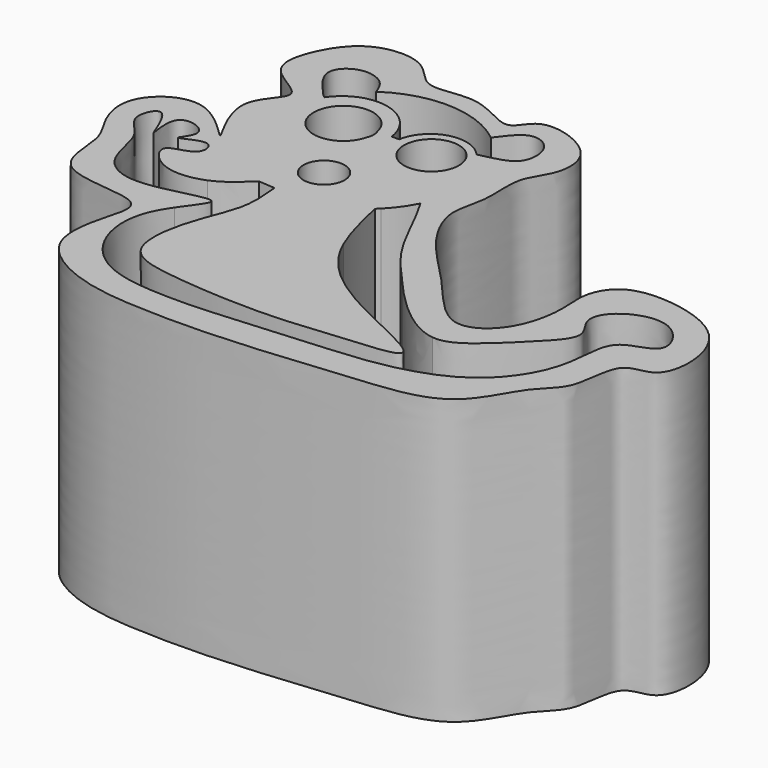
from build123d import *

# Parameters (mm, degrees)
F0_R     = 3.7205580231
F1_DEPTH = 51.562


with BuildPart() as f1:
    # F0 (on Top) → F1 (new body)
    with BuildSketch(Plane.XY):
        with BuildLine():
            add(Edge.make_bspline(
                [(-53.0351996422, 40.0811992586), (-53.3079930687, 41.6627953679), (-60.7647197567, 44.1354743978), (-59.1255177726, 52.4056801186), (-53.9738105286, 59.9405136718), (-43.6820680314, 60.0552836973), (-40.0768432819, 52.8134528274), (-30.922173083, 56.6842073685), (-22.4287718601, 49.6258780063), (-20.555433276, 57.2186201881), (-8.0154700964, 53.1735527396), (-7.9074828777, 44.5223918176), (-12.1257390745, 40.114923321), (-10.7256442044, 31.933104297), (-13.5341011998, 25.6774370624), (-8.5652531319, 16.3662428058), (-0.0531398385, 8.862949751), (8.2077255005, -2.4517748861), (16.5242775456, 2.6540873778), (18.6817624376, 12.0345401673), (17.4626842494, 17.7274123298), (20.6284477431, 24.0450881696), (30.6198326835, 24.2634316934), (39.9883133501, 20.6347344654), (43.274263606, 12.4930502219), (41.8209757823, 4.373088916), (34.4557856792, 5.3826149304), (35.1162405235, -5.4890850104), (29.2679840475, -8.9956139239), (24.7245789247, -21.1012100778), (8.5716456517, -22.3660177487), (-3.2073427267, -23.673208758), (-17.0097819532, -24.6958343574), (-27.8201507989, -24.6594358256), (-40.6695843247, -23.820251083), (-51.9653752301, -17.0200309695), (-50.4154986842, -6.6540089959), (-47.0885578266, 2.3917477436), (-66.4204916011, 0.0746272617), (-65.0768362054, 12.6106814261), (-68.7260787409, 16.8312978332), (-71.4451206704, 25.4892643605), (-60.6602210105, 33.1244068312), (-49.112760512, 18.8797609199), (-59.7521417466, 34.36020266), (-52.7621453219, 38.4980905445), (-53.0351996422, 40.0811992586)],
                knots=[0, 0, 0, 0, 0.0210227239, 0.0415498789, 0.0644000682, 0.0870516541, 0.1064951093, 0.129047416, 0.1514029912, 0.1678357279, 0.1925133649, 0.2131914357, 0.2315774148, 0.2528958574, 0.2725256217, 0.2962058086, 0.3233948157, 0.3502333972, 0.3708847816, 0.3943700022, 0.4129475644, 0.4314604615, 0.4548624528, 0.4788890461, 0.5011629669, 0.5210807734, 0.5382113528, 0.5607203848, 0.5804368125, 0.606432177, 0.6361158369, 0.6634705602, 0.6917741726, 0.7173460798, 0.7451067546, 0.7712430171, 0.7953524467, 0.8146494037, 0.8431599135, 0.8666451338, 0.8851189078, 0.9065051395, 0.9308580695, 0.9545133683, 0.9789571704, 1, 1, 1, 1], degree=3))
        make_face()
        with BuildLine():
            add(Edge.make_bspline(
                [(-21.0652948492, 20.6782598491), (-21.670172812, 20.639156422), (-21.7699233734, 20.2162934835), (-21.7458119728, 20.0338150913)],
                knots=[0.8847102512, 0.8847102512, 0.8847102512, 0.8847102512, 0.9803485, 0.9803485, 0.9803485, 0.9803485], degree=3))
            ThreePointArc((-21.0652948492, 20.6782598491), (-19.1925492315, 22.8925325451), (-17.6995540947, 25.3787234554))
            add(Edge.make_bspline(
                [(-8.1258436749, 8.8725080124), (-8.9507770078, 9.8625538653), (-11.8076923951, 13.5529828734), (-14.9203133764, 20.5039164014), (-16.8647921862, 23.9151210734), (-17.6995540947, 25.3787234554)],
                knots=[0.936730527, 0.936730527, 0.936730527, 0.936730527, 0.948494633, 0.9779000116, 1, 1, 1, 1], degree=3))
            add(Edge.make_bspline(
                [(-8.1258436749, 8.8725080124), (-6.9920288455, 7.5914053785), (-5.8582140161, 6.3103027445), (-4.7243991867, 5.0292001106)],
                knots=[0, 0, 0, 0, 5.1323328258, 5.1323328258, 5.1323328258, 5.1323328258], degree=3))
            add(Edge.make_bspline(
                [(9.2964004725, -5.6388000958), (6.2140361423, -5.3139568809), (-0.4758535739, 0.0377445161), (-3.1854275389, 3.3122390614), (-4.7243991867, 5.0292001106)],
                knots=[0.8640116613, 0.8640116613, 0.8640116613, 0.8640116613, 0.8951731635, 0.9199974846, 0.9199974846, 0.9199974846, 0.9199974846], degree=3))
            add(Edge.make_bspline(
                [(-44.1327011496, 2.6484160648), (-44.7130309574, 1.8048856406), (-47.6946083402, -2.927021188), (-46.8772518965, -11.6007203583), (-39.5802529159, -18.6266633144), (-28.3429017795, -19.591076178), (-18.1242244322, -19.144415426), (-6.9103865804, -18.0520208922), (4.7211664853, -17.4405127728), (13.9368833116, -15.7759420728), (23.8112421331, -11.3932618369), (30.3389740044, -0.7257155667), (28.9709345734, 10.3098746354), (39.2162281551, 10.6255935235), (33.8249627001, 20.1168201293), (24.5686551298, 17.1746113113), (22.2539715483, 11.9137811577), (26.7972968019, 7.9772485427), (21.1542360401, 2.2425014104), (16.0200417627, -2.9179627405), (11.7632185561, -5.8987723219), (9.2964004725, -5.6388000958)],
                knots=[0.3585684754, 0.3585684754, 0.3585684754, 0.3585684754, 0.3659479306, 0.3974689583, 0.4260715846, 0.4571624421, 0.4875914142, 0.5193796367, 0.5515918337, 0.5804502736, 0.6108726721, 0.6438200053, 0.672548465, 0.6962237578, 0.7206702006, 0.748010088, 0.7683723479, 0.7881144061, 0.8123813661, 0.8390730918, 0.8640116613, 0.8640116613, 0.8640116613, 0.8640116613], degree=3))
            add(Edge.make_bspline(
                [(-49.0828990199, 6.1701741385), (-49.177863489, 4.040428207), (-47.197859123, 2.9614294526), (-44.13270115, 2.6484160654)],
                knots=[0.0841406615, 0.0841406615, 0.0841406615, 0.0841406615, 0.208246285, 0.208246285, 0.208246285, 0.208246285], degree=3))
            add(Edge.make_bspline(
                [(-45.71999982, 12.0395999402), (-48.2095024269, 11.0006678158), (-53.7802194274, 10.5093334281), (-58.6217302771, 16.9809530467), (-51.186861328, 16.9659773531), (-52.1172615159, 22.6049918831), (-59.260802502, 17.953520738), (-53.6590125511, 23.3854970332), (-62.6446993243, 26.277051321), (-59.5639044419, 14.4067842249), (-63.6375573492, 27.3151683753), (-66.9947393471, 20.1703294936), (-61.4699964034, 17.1271549744), (-61.3142437426, 8.4281658926), (-55.8384577489, 5.0155903157), (-50.3902321248, 5.8993125354), (-49.0828990199, 6.1701741385)],
                knots=[0.0256288773, 0.0256288773, 0.0256288773, 0.0256288773, 0.0524870758, 0.0732332952, 0.0938749966, 0.1097169476, 0.1296254117, 0.1467479568, 0.1673048843, 0.1888353489, 0.2125106443, 0.2303278097, 0.2524804134, 0.2787225334, 0.3057488565, 0.3143296922, 0.3143296922, 0.3143296922, 0.3143296922], degree=3))
            add(Edge.make_bspline(
                [(-39.7831306216, 16.380742902), (-41.56390775, 14.7159485647), (-43.3444437298, 13.0309793139), (-45.71999982, 12.0395999402)],
                knots=[0, 0, 0, 0, 0.0256288773, 0.0256288773, 0.0256288773, 0.0256288773], degree=3))
            add(Edge.make_bspline(
                [(-39.7831306216, 16.380742902), (-38.95093334, 16.2972918142), (-38.134915658, 16.2371630687), (-37.335459951, 16.2009078471)],
                knots=[0, 0, 0, 0, 2.0774208338, 2.0774208338, 2.0774208338, 2.0774208338], degree=3))
            add(Edge.make_bspline(
                [(-37.335459951, 16.2009078471), (-31.0549759584, 15.916088642), (-25.796629976, 17.1046466153), (-21.7458119642, 20.0338150896)],
                knots=[2.0774208338, 2.0774208338, 2.0774208338, 2.0774208338, 18.3975348551, 18.3975348551, 18.3975348551, 18.3975348551], degree=3))
        make_face(mode=Mode.SUBTRACT)
        with Locations((-34.2900007963, 24.2315996438)):
            Circle(F0_R, mode=Mode.SUBTRACT)
        with BuildLine():
            ThreePointArc((-36.3116717652, 36.4814959466), (-46.971085664, 37.8051259579), (-36.2804545776, 38.8470031321))
            add(Edge.make_bspline(
                [(-36.2804545776, 38.8470031321), (-36.2042632894, 38.638003094), (-36.0421633968, 38.1933474837), (-36.013318579, 37.2966688863), (-36.2123204756, 36.7529476575), (-36.3116717652, 36.4814959466)],
                knots=[0, 0, 0, 0, 0.307532383, 0.6542869592, 1, 1, 1, 1], degree=3))
        make_face(mode=Mode.SUBTRACT)
        with BuildLine():
            ThreePointArc((-20.7269751995, 37.8729701042), (-30.0915433108, 35.5184298259), (-22.954191543, 42.0220600103))
            ThreePointArc((-22.954191543, 42.0220600103), (-21.3189790012, 40.2275103826), (-20.7269751995, 37.8729701042))
        make_face(mode=Mode.SUBTRACT)
        with BuildLine():
            ThreePointArc((-33.7017707591, 38.8470031321), (-39.999476926, 45.7439636175), (-48.6812743523, 42.3007731858))
            add(Edge.make_bspline(
                [(-49.2198829041, 42.7281072575), (-49.0385020241, 42.5844299812), (-48.8626552323, 42.4444504621), (-48.6812743523, 42.3007731858)],
                knots=[0, 0, 0, 0, 0.687541694, 0.687541694, 0.687541694, 0.687541694], degree=3))
            add(Edge.make_bspline(
                [(-49.2198829041, 42.7281072575), (-51.19934658, 44.8979233113), (-54.7239489701, 48.7439745563), (-50.1221749988, 52.81542629), (-45.2801795053, 51.5125545977), (-44.4254927385, 49.2654049663), (-44.0268645913, 48.2185372916)],
                knots=[0, 0, 0, 0, 0.310725073, 0.5499326634, 0.79062154, 1, 1, 1, 1], degree=3))
            ThreePointArc((-44.0268645913, 48.2185372916), (-33.1420930224, 51.3687844299), (-22.5308552567, 47.3933671914))
            add(Edge.make_bspline(
                [(-22.5308552567, 47.3933671914), (-21.2095190932, 49.205980475), (-18.7721682592, 52.552915334), (-13.7470974395, 50.0324472001), (-13.8185248481, 43.9096057901), (-16.9020924696, 43.0581948555), (-18.3954862509, 42.6449623371)],
                knots=[0, 0, 0, 0, 0.2768007406, 0.5090744039, 0.7627286351, 1, 1, 1, 1], degree=3))
            add(Edge.make_bspline(
                [(-18.3954862509, 42.6449623371), (-19.1555240256, 42.4677094098), (-19.9155618003, 42.2904564826), (-20.675599575, 42.1132035553)],
                knots=[0, 0, 0, 0, 2.341299676, 2.341299676, 2.341299676, 2.341299676], degree=3))
            add(Edge.make_bspline(
                [(-20.675599575, 42.1132035553), (-20.7297600417, 42.0839673312), (-20.7802752843, 42.0578559737), (-20.8344357509, 42.0286197495)],
                knots=[0, 0, 0, 0, 0.1799537468, 0.1799537468, 0.1799537468, 0.1799537468], degree=3))
            ThreePointArc((-20.8344357509, 42.0286197495), (-20.8671966944, 42.0665437034), (-20.9002447034, 42.1042177634))
            ThreePointArc((-20.9002447034, 42.1042177634), (-27.6501958711, 44.0808092286), (-32.3487092883, 38.8470031321))
            Line((-32.3487092883, 38.8470031321), (-33.7017707591, 38.8470031321))
        make_face(mode=Mode.SUBTRACT)
        with BuildLine():
            add(Edge.make_bspline(
                [(-38.8865054324, 2.7137341923), (-39.2013483841, 1.8508518548), (-40.6857275806, -2.479034825), (-41.857395368, -12.156175759), (-30.2869064904, -14.3210148671), (-13.4186121607, -15.3017300236), (-1.8057579388, -13.7083720265), (15.1351427548, -12.8048451743), (-7.3018340252, -4.1578341465), (-15.5277854797, 2.920156624), (-18.0961822011, 8.0444989939), (-18.4368261233, 8.8112696576)],
                knots=[0.141118669, 0.141118669, 0.141118669, 0.141118669, 0.1655386981, 0.2585924292, 0.3477026087, 0.4665688636, 0.573696851, 0.6603811929, 0.7756371935, 0.8916603721, 0.9113790023, 0.9113790023, 0.9113790023, 0.9113790023], degree=3))
            add(Edge.make_bspline(
                [(-38.8865054322, 2.7137341917), (-32.1377612072, 3.3669214959), (-23.6097595892, 5.891801251), (-18.4368261233, 8.8112696576)],
                knots=[0.2698570737, 0.2698570737, 0.2698570737, 0.2698570737, 0.4846901848, 0.4846901848, 0.4846901848, 0.4846901848], degree=3))
        make_face()
        with BuildLine():
            add(Edge.make_bspline(
                [(-18.4368261233, 8.8112696576), (-19.9677744688, 12.2573498677), (-20.8431582774, 16.1554617481), (-21.718542086, 20.0535736285)],
                knots=[0.9113790023, 0.9113790023, 0.9113790023, 0.9113790023, 1, 1, 1, 1], degree=3))
            add(Edge.make_bspline(
                [(-21.7458119728, 20.0338150913), (-21.7456147196, 20.0323222517), (-21.7404521603, 19.9952311482), (-21.7301917205, 19.9685048959), (-21.718542086, 20.0535736285)],
                knots=[0.9803485, 0.9803485, 0.9803485, 0.9803485, 0.981130908, 1, 1, 1, 1], degree=3))
            add(Edge.make_bspline(
                [(-37.335459951, 16.2009078471), (-31.0549759584, 15.916088642), (-25.796629976, 17.1046466153), (-21.7458119642, 20.0338150896)],
                knots=[2.0774208338, 2.0774208338, 2.0774208338, 2.0774208338, 18.3975348551, 18.3975348551, 18.3975348551, 18.3975348551], degree=3))
            add(Edge.make_bspline(
                [(-37.335459951, 16.2009078471), (-37.2443888599, 16.1912422791), (-37.0556519801, 16.1701375357), (-36.8026544835, 16.1415062215)],
                knots=[0, 0, 0, 0, 0.8497261991, 0.8497261991, 0.8497261991, 0.8497261991], degree=3))
            add(Edge.make_bspline(
                [(-36.8026544977, 16.1415062173), (-36.5705358682, 13.7622348174), (-36.1455330702, 9.4005594138), (-38.0597561396, 4.9795856544), (-38.8865054324, 2.7137341923)],
                knots=[3.10934e-05, 3.10934e-05, 3.10934e-05, 3.10934e-05, 0.0769938675, 0.141118669, 0.141118669, 0.141118669, 0.141118669], degree=3))
            add(Edge.make_bspline(
                [(-38.8865054322, 2.7137341917), (-32.1377612072, 3.3669214959), (-23.6097595892, 5.891801251), (-18.4368261233, 8.8112696576)],
                knots=[0.2698570737, 0.2698570737, 0.2698570737, 0.2698570737, 0.4846901848, 0.4846901848, 0.4846901848, 0.4846901848], degree=3))
        make_face()
        with BuildLine():
            add(Edge.make_bspline(
                [(-49.0828990199, 6.1701741385), (-49.177863489, 4.040428207), (-47.197859123, 2.9614294526), (-44.13270115, 2.6484160654)],
                knots=[0.0841406615, 0.0841406615, 0.0841406615, 0.0841406615, 0.208246285, 0.208246285, 0.208246285, 0.208246285], degree=3))
            add(Edge.make_bspline(
                [(-49.0828990199, 6.1701741385), (-45.4599015722, 6.9208098354), (-38.8001175875, 9.1444431667), (-42.5237941185, 4.9870207894), (-44.1327011496, 2.6484160648)],
                knots=[0.3143296922, 0.3143296922, 0.3143296922, 0.3143296922, 0.3381096654, 0.3585684754, 0.3585684754, 0.3585684754, 0.3585684754], degree=3))
        make_face()
        with BuildLine():
            add(Edge.make_bspline(
                [(-21.7458119642, 20.0338150896), (-21.7367159155, 20.0403924917), (-21.7276259554, 20.0469786703), (-21.718542086, 20.0535736285)],
                knots=[18.3975348551, 18.3975348551, 18.3975348551, 18.3975348551, 18.4341814167, 18.4341814167, 18.4341814167, 18.4341814167], degree=3))
            ThreePointArc((-21.718542086, 20.0535736285), (-21.3879982127, 20.3618172476), (-21.0652948492, 20.6782598491))
            add(Edge.make_bspline(
                [(-21.0652948492, 20.6782598491), (-21.670172812, 20.639156422), (-21.7699233734, 20.2162934835), (-21.7458119728, 20.0338150913)],
                knots=[0.8847102512, 0.8847102512, 0.8847102512, 0.8847102512, 0.9803485, 0.9803485, 0.9803485, 0.9803485], degree=3))
        make_face()
        with BuildLine():
            add(Edge.make_bspline(
                [(-21.7458119728, 20.0338150913), (-21.7456147196, 20.0323222517), (-21.7404521603, 19.9952311482), (-21.7301917205, 19.9685048959), (-21.718542086, 20.0535736285)],
                knots=[0.9803485, 0.9803485, 0.9803485, 0.9803485, 0.981130908, 1, 1, 1, 1], degree=3))
            add(Edge.make_bspline(
                [(-21.7458119642, 20.0338150896), (-21.7367159155, 20.0403924917), (-21.7276259554, 20.0469786703), (-21.718542086, 20.0535736285)],
                knots=[18.3975348551, 18.3975348551, 18.3975348551, 18.3975348551, 18.4341814167, 18.4341814167, 18.4341814167, 18.4341814167], degree=3))
        make_face()
    extrude(amount=F1_DEPTH)


solid = f1.part
